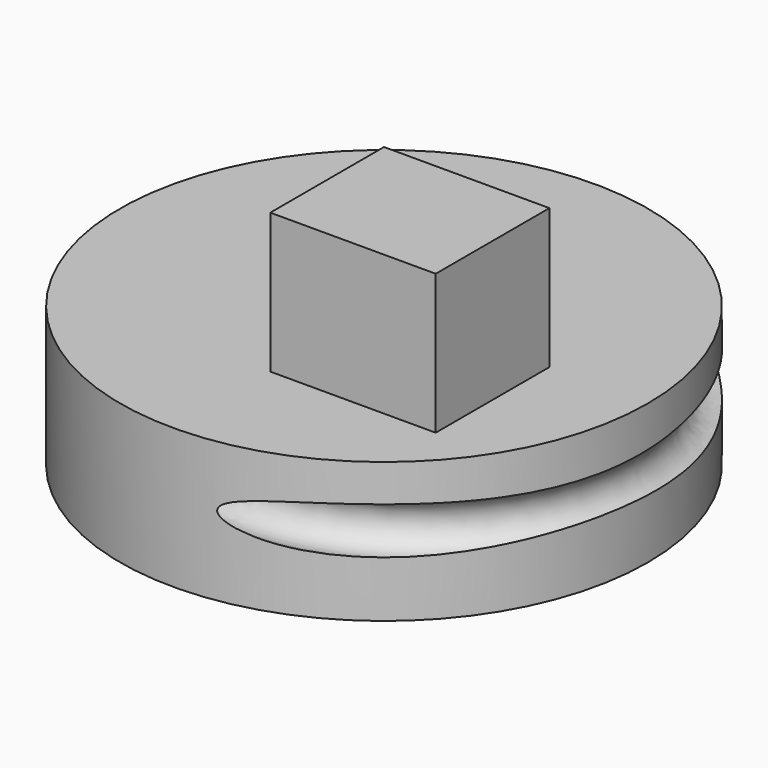
from build123d import *

# Parameters (mm, degrees)
F1_R     = 47.8906341697
F3_DEPTH = 25.4
F2_W     = 30.0199426711
F2_H     = 25.7944688201
F4_DEPTH = 25.4
F7_R     = 4.2429445986


# Not quite as in the source:
# - a feature of the source that left no trace in its solid (it failed there, or was rolled back) is left out


with BuildPart() as f3:
    # F1 (on Top) → F3 (new body)
    with BuildSketch(Plane.XY):
        Circle(F1_R)
    extrude(amount=F3_DEPTH)

    # F2 (on offset) → F4 (join)
    with BuildSketch(Plane.XY.offset(50.8)):
        with Locations((15.0099713355, -12.89723441)):
            Rectangle(F2_W, F2_H)
    extrude(amount=-F4_DEPTH)

    # F8: sweep along a path in F6
    with BuildLine(Plane.XY.offset(12.7)) as f8_path:
        CenterArc((9.0787773952, -2.0044676494), 44.2959341801, 0, 360)
    # F7 (on Front) → F8 (sweep, cut)
    with BuildSketch(Plane.XZ):
        with Locations((50.1028448343, 14.4018204883)):
            Circle(F7_R)
    sweep(path=f8_path.line, mode=Mode.SUBTRACT)


solid = f3.part
